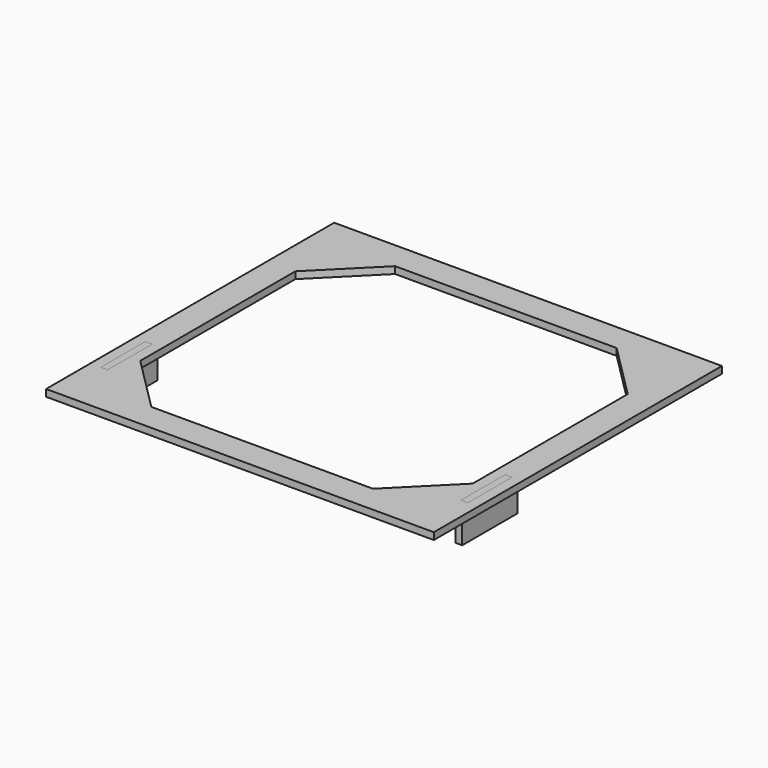
from build123d import *

# Parameters (mm, degrees)
F0_W     = 355.6
F0_H     = 330.2
F0_W_2   = 304.8
F0_H_2   = 279.4
F0_W_3   = 6.35
F0_H_3   = 6.35
F1_DEPTH = 6.35
F2_SIZE  = 50.8
F0_H_4   = 50.8
F3_DEPTH = 6.35
F4_DEPTH = 25.4


with BuildPart() as f1:
    # F0 (on Top) → F1 (new body)
    with BuildSketch(Plane.XY):
        with Locations((177.8, 165.1)):
            Rectangle(F0_W, F0_H)
        Polygon((9.525, 44.45), (9.525, 50.8), (9.525, 101.6), (9.525, 107.95), (15.875, 107.95), (15.875, 101.6), (15.875, 50.8), (15.875, 44.45), align=None, mode=Mode.SUBTRACT)
        Polygon((346.075, 101.6), (346.075, 50.8), (346.075, 44.45), (339.725, 44.45), (339.725, 50.8), (339.725, 101.6), (339.725, 107.95), (346.075, 107.95), align=None, mode=Mode.SUBTRACT)
        with Locations((177.8, 165.1)):
            Rectangle(F0_W_2, F0_H_2, mode=Mode.SUBTRACT)
        with Locations((12.7, 47.625)):
            Rectangle(F0_W_3, F0_H_3)
        with Locations((342.9, 47.625)):
            Rectangle(F0_W_3, F0_H_3)
        with Locations((342.9, 104.775)):
            Rectangle(F0_W_3, F0_H_3)
        with Locations((12.7, 104.775)):
            Rectangle(F0_W_3, F0_H_3)
    extrude(amount=F1_DEPTH)

    # F2
    f2_edges = [f1.edges().sort_by_distance(p)[0] for p in [
        (25.4, 304.8, 3.175),
        (25.4, 25.4, 3.175),
        (330.2, 25.4, 3.175),
        (330.2, 304.8, 3.175),
    ]]
    chamfer(f2_edges, length=F2_SIZE)


with BuildPart() as f3:
    # F0 (on Top) → F3 (new body, through all)
    with BuildSketch(Plane.XY):
        with Locations((12.7, 76.2)):
            Rectangle(F0_W_3, F0_H_4)
    extrude(amount=F3_DEPTH)

    # F0 (on Top) → F4 (join)
    with BuildSketch(Plane.XY):
        with Locations((12.7, 47.625)):
            Rectangle(F0_W_3, F0_H_3)
        with Locations((12.7, 76.2)):
            Rectangle(F0_W_3, F0_H_4)
        with Locations((12.7, 104.775)):
            Rectangle(F0_W_3, F0_H_3)
    extrude(amount=-F4_DEPTH)


with BuildPart() as f3b:
    # F0 (on Top) → F3, piece 2 (new body, through all)
    with BuildSketch(Plane.XY):
        with Locations((342.9, 76.2)):
            Rectangle(F0_W_3, F0_H_4)
    extrude(amount=F3_DEPTH)

    # F0 (on Top) → F4, piece 2 (join)
    with BuildSketch(Plane.XY):
        with Locations((342.9, 47.625)):
            Rectangle(F0_W_3, F0_H_3)
        with Locations((342.9, 76.2)):
            Rectangle(F0_W_3, F0_H_4)
        with Locations((342.9, 104.775)):
            Rectangle(F0_W_3, F0_H_3)
    extrude(amount=-F4_DEPTH)


solid = Compound([f1.part, f3.part, f3b.part])
